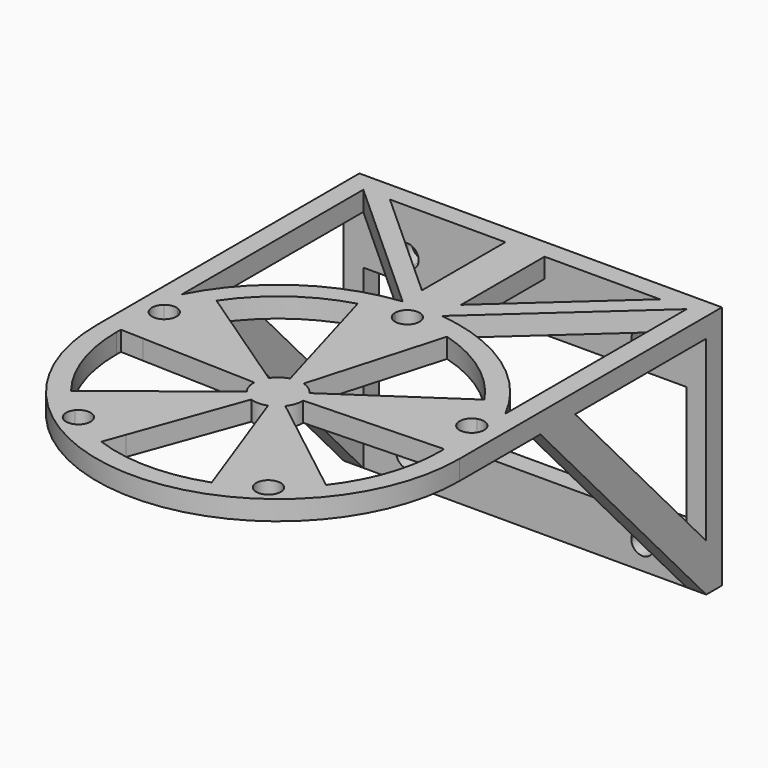
from build123d import *

# Parameters (mm, degrees)
F1_DEPTH = 4
F3_DEPTH = 4
F5_DEPTH = 4
F6_W     = 4
F6_H     = 26
F6_H_2   = 10
F7_DEPTH = 4


with BuildPart() as f1:
    # F0 (on Top) → F1 (new body)
    with BuildSketch(Plane.XY):
        with BuildLine():
            ThreePointArc((-2.498205853, 32.9053030303), (-0.0473569821, 35.499551423), (2.5, 33))
            ThreePointArc((2.5, 33), (2.499551423, 32.9526430179), (2.498205853, 32.9053030303))
            ThreePointArc((2.498205853, 32.9053030303), (5.8372772609, 32.4796273713), (9.1156141969, 31.7160145323))
            ThreePointArc((9.1156141969, 31.7160145323), (19.3969133257, 26.6975608144), (27.3468425908, 18.4702517664))
            ThreePointArc((27.3468425908, 18.4702517664), (29.0861433838, 15.5883374051), (30.5228148036, 12.544232797))
            ThreePointArc((30.5228148036, 12.544232797), (31.8205738268, 12.6592996005), (33, 12.1057901124))
            Line((33, 12.1057901124), (33, 16.7332005307))
            ThreePointArc((33, 16.7332005307), (21.0416278254, 30.4343539188), (4, 36.7831483155))
            ThreePointArc((4, 36.7831483155), (0, 37), (-4, 36.7831483155))
            ThreePointArc((-4, 36.7831483155), (-21.0416278254, 30.4343539188), (-33, 16.7332005307))
            Line((-33, 16.7332005307), (-33, 12.1057901124))
            ThreePointArc((-33, 12.1057901124), (-31.8205738268, 12.6592996005), (-30.5228148036, 12.544232797))
            ThreePointArc((-30.5228148036, 12.544232797), (-29.0861433838, 15.5883374051), (-27.3468425908, 18.4702517664))
            ThreePointArc((-27.3468425908, 18.4702517664), (-19.3969133257, 26.6975608144), (-9.1156141969, 31.7160145323))
            ThreePointArc((-9.1156141969, 31.7160145323), (-5.8372772609, 32.4796273713), (-2.498205853, 32.9053030303))
        make_face()
        with BuildLine():
            ThreePointArc((2.498205853, 32.9053030303), (0, 30.5), (-2.498205853, 32.9053030303))
            ThreePointArc((-2.498205853, 32.9053030303), (-5.8372772609, 32.4796273713), (-9.1156141969, 31.7160145323))
            Line((-9.1156141969, 31.7160145323), (-7.8462162594, 27.2993902036))
            Line((-7.8462162594, 27.2993902036), (-1.3811536662, 4.8054567473))
            ThreePointArc((-1.3811536662, 4.8054567473), (0, 5), (1.3811536662, 4.8054567473))
            Line((1.3811536662, 4.8054567473), (7.8462162594, 27.2993902036))
            Line((7.8462162594, 27.2993902036), (9.1156141969, 31.7160145323))
            ThreePointArc((9.1156141969, 31.7160145323), (5.8372772609, 32.4796273713), (2.498205853, 32.9053030303))
        make_face()
        with BuildLine():
            Line((-4.1434609986, 2.7985229949), (-27.3468425908, 18.4702517664))
            ThreePointArc((-27.3468425908, 18.4702517664), (-29.0861433838, 15.5883374051), (-30.5228148036, 12.544232797))
            ThreePointArc((-30.5228148036, 12.544232797), (-29.3348497225, 11.6284476748), (-28.8848650377, 10.1975608144))
            ThreePointArc((-28.8848650377, 10.1975608144), (-29.8773529706, 8.2032169705), (-32.0667909317, 7.7923628859))
            ThreePointArc((-32.0667909317, 7.7923628859), (-32.6937791328, 4.4851762523), (-32.9806019929, 1.1313232023))
            Line((-32.9806019929, 1.1313232023), (-28.3878771097, 0.9737804072))
            Line((-28.3878771097, 0.9737804072), (-4.997060908, 0.1714126064))
            ThreePointArc((-4.997060908, 0.1714126064), (-4.7552825815, 1.5450849719), (-4.1434609986, 2.7985229949))
        make_face()
        with BuildLine():
            ThreePointArc((30.5228148036, 12.544232797), (29.0861433838, 15.5883374051), (27.3468425908, 18.4702517664))
            Line((27.3468425908, 18.4702517664), (23.5386487783, 15.8981706108))
            Line((23.5386487783, 15.8981706108), (4.1434609986, 2.7985229949))
            ThreePointArc((4.1434609986, 2.7985229949), (4.7552825815, 1.5450849719), (4.997060908, 0.1714126064))
            Line((4.997060908, 0.1714126064), (32.9806019929, 1.1313232023))
            ThreePointArc((32.9806019929, 1.1313232023), (32.6937791328, 4.4851762523), (32.0667909317, 7.7923628859))
            ThreePointArc((32.0667909317, 7.7923628859), (29.007223747, 9.4250183284), (30.5228148036, 12.544232797))
        make_face()
        with BuildLine():
            ThreePointArc((1.3811536662, 4.8054567473), (0, 5), (-1.3811536662, 4.8054567473))
            Line((-1.3811536662, 4.8054567473), (0, 0))
            Line((0, 0), (1.3811536662, 4.8054567473))
        make_face()
        with BuildLine():
            Line((0, 0), (-1.3811536662, 4.8054567473))
            ThreePointArc((-1.3811536662, 4.8054567473), (-2.9389262615, 4.0450849719), (-4.1434609986, 2.7985229949))
            Line((-4.1434609986, 2.7985229949), (0, 0))
        make_face()
        with BuildLine():
            Line((0, 0), (-4.1434609986, 2.7985229949))
            ThreePointArc((-4.1434609986, 2.7985229949), (-4.7552825815, 1.5450849719), (-4.997060908, 0.1714126064))
            Line((-4.997060908, 0.1714126064), (0, 0))
        make_face()
        with BuildLine():
            ThreePointArc((4.1434609986, 2.7985229949), (2.9389262615, 4.0450849719), (1.3811536662, 4.8054567473))
            Line((1.3811536662, 4.8054567473), (0, 0))
            Line((0, 0), (4.1434609986, 2.7985229949))
        make_face()
        with BuildLine():
            Line((-1.7071998188, -4.6995179305), (0, 0))
            Line((0, 0), (-3.9419533944, -3.0758744182))
            ThreePointArc((-3.9419533944, -3.0758744182), (-2.9389262615, -4.0450849719), (-1.7071998188, -4.6995179305))
        make_face()
        with BuildLine():
            Line((-3.9419533944, -3.0758744182), (0, 0))
            Line((0, 0), (-4.997060908, 0.1714126064))
            ThreePointArc((-4.997060908, 0.1714126064), (-4.7552825815, -1.5450849719), (-3.9419533944, -3.0758744182))
        make_face()
        with BuildLine():
            Line((3.9419533944, -3.0758744182), (0, 0))
            Line((0, 0), (1.7071998188, -4.6995179305))
            ThreePointArc((1.7071998188, -4.6995179305), (2.9389262615, -4.0450849719), (3.9419533944, -3.0758744182))
        make_face()
        with BuildLine():
            Line((1.7071998188, -4.6995179305), (0, 0))
            Line((0, 0), (-1.7071998188, -4.6995179305))
            ThreePointArc((-1.7071998188, -4.6995179305), (0, -5), (1.7071998188, -4.6995179305))
        make_face()
        with BuildLine():
            Line((4.1434609986, 2.7985229949), (0, 0))
            Line((0, 0), (4.997060908, 0.1714126064))
            ThreePointArc((4.997060908, 0.1714126064), (4.7552825815, 1.5450849719), (4.1434609986, 2.7985229949))
        make_face()
        with BuildLine():
            Line((4.997060908, 0.1714126064), (0, 0))
            Line((0, 0), (3.9419533944, -3.0758744182))
            ThreePointArc((3.9419533944, -3.0758744182), (4.7280951224, -1.6263814171), (5, 0))
            ThreePointArc((5, 0), (4.999265173, 0.0857189009), (4.997060908, 0.1714126064))
        make_face()
        with BuildLine():
            ThreePointArc((-33, 8.2893315164), (-33.8848650377, 10.1975608144), (-33, 12.1057901124))
            Line((-33, 12.1057901124), (-33, 16.7332005307))
            ThreePointArc((-33, 16.7332005307), (-35.9861084309, 8.602325267), (-37, 0))
            ThreePointArc((-37, 0), (0, -37), (37, 0))
            ThreePointArc((37, 0), (35.9861084309, 8.602325267), (33, 16.7332005307))
            Line((33, 16.7332005307), (33, 12.1057901124))
            ThreePointArc((33, 12.1057901124), (33.6528859157, 11.2492648113), (33.8848650377, 10.1975608144))
            ThreePointArc((33.8848650377, 10.1975608144), (33.6528859157, 9.1458568174), (33, 8.2893315164))
            Line((33, 8.2893315164), (33, 0))
            ThreePointArc((33, 0), (31.2054278075, -10.7341173531), (26.0168924031, -20.3007711599))
            ThreePointArc((26.0168924031, -20.3007711599), (23.8135024738, -22.8455050268), (21.3623428339, -25.152540799))
            ThreePointArc((21.3623428339, -25.152540799), (21.759493882, -25.8801177799), (21.8969133257, -26.6975608144))
            ThreePointArc((21.8969133257, -26.6975608144), (20.1242780272, -29.0894095953), (17.3201608529, -28.0893579142))
            ThreePointArc((17.3201608529, -28.0893579142), (14.3685894638, -29.7076360019), (11.2675188041, -31.016818341))
            ThreePointArc((11.2675188041, -31.016818341), (0, -33), (-11.2675188041, -31.016818341))
            ThreePointArc((-11.2675188041, -31.016818341), (-14.3685894638, -29.7076360019), (-17.3201608529, -28.0893579142))
            ThreePointArc((-17.3201608529, -28.0893579142), (-20.8663764564, -28.7201033003), (-21.3623428339, -25.152540799))
            ThreePointArc((-21.3623428339, -25.152540799), (-23.8135024738, -22.8455050268), (-26.0168924031, -20.3007711599))
            ThreePointArc((-26.0168924031, -20.3007711599), (-31.2054278075, -10.7341173531), (-33, 0))
            Line((-33, 0), (-33, 8.2893315164))
        make_face()
        with BuildLine():
            ThreePointArc((-32.9806019929, 1.1313232023), (-32.6937791328, 4.4851762523), (-32.0667909317, 7.7923628859))
            ThreePointArc((-32.0667909317, 7.7923628859), (-32.5599678414, 7.9909495208), (-33, 8.2893315164))
            Line((-33, 8.2893315164), (-33, 0))
            ThreePointArc((-33, 0), (-32.9951501418, 0.565744746), (-32.9806019929, 1.1313232023))
        make_face()
        with BuildLine():
            ThreePointArc((33, 8.2893315164), (32.5599678414, 7.9909495208), (32.0667909317, 7.7923628859))
            ThreePointArc((32.0667909317, 7.7923628859), (32.6937791328, 4.4851762523), (32.9806019929, 1.1313232023))
            ThreePointArc((32.9806019929, 1.1313232023), (32.9951501418, 0.565744746), (33, 0))
            Line((33, 0), (33, 8.2893315164))
        make_face()
        with BuildLine():
            ThreePointArc((-1.7071998188, -4.6995179305), (-2.9389262615, -4.0450849719), (-3.9419533944, -3.0758744182))
            Line((-3.9419533944, -3.0758744182), (-26.0168924031, -20.3007711599))
            ThreePointArc((-26.0168924031, -20.3007711599), (-23.8135024738, -22.8455050268), (-21.3623428339, -25.152540799))
            ThreePointArc((-21.3623428339, -25.152540799), (-18.5794702912, -24.334980258), (-16.8969133257, -26.6975608144))
            ThreePointArc((-16.8969133257, -26.6975608144), (-17.0050645447, -27.4249255159), (-17.3201608529, -28.0893579142))
            ThreePointArc((-17.3201608529, -28.0893579142), (-14.3685894638, -29.7076360019), (-11.2675188041, -31.016818341))
            Line((-11.2675188041, -31.016818341), (-9.6984566628, -26.6975608144))
            Line((-9.6984566628, -26.6975608144), (-1.7071998188, -4.6995179305))
        make_face()
        with BuildLine():
            ThreePointArc((3.9419533944, -3.0758744182), (2.9389262615, -4.0450849719), (1.7071998188, -4.6995179305))
            Line((1.7071998188, -4.6995179305), (11.2675188041, -31.016818341))
            ThreePointArc((11.2675188041, -31.016818341), (14.3685894638, -29.7076360019), (17.3201608529, -28.0893579142))
            ThreePointArc((17.3201608529, -28.0893579142), (17.9274501949, -24.6750183284), (21.3623428339, -25.152540799))
            ThreePointArc((21.3623428339, -25.152540799), (23.8135024738, -22.8455050268), (26.0168924031, -20.3007711599))
            Line((26.0168924031, -20.3007711599), (22.3939012537, -17.4737804072))
            Line((22.3939012537, -17.4737804072), (3.9419533944, -3.0758744182))
        make_face()
        with BuildLine():
            ThreePointArc((-37, 0), (-35.9861084309, 8.602325267), (-33, 16.7332005307))
            Line((-33, 16.7332005307), (-33, 63))
            Line((-33, 63), (-27.5608655065, 63))
            Line((-27.5608655065, 63), (-4, 63))
            Line((-4, 63), (0, 63))
            Line((0, 63), (4, 63))
            Line((4, 63), (27.5608655065, 63))
            Line((27.5608655065, 63), (33, 63))
            Line((33, 63), (33, 16.7332005307))
            ThreePointArc((33, 16.7332005307), (35.9861084309, 8.602325267), (37, 0))
            Line((37, 0), (37, 67))
            Line((37, 67), (0, 67))
            Line((0, 67), (-37, 67))
            Line((-37, 67), (-37, 0))
        make_face()
        Polygon((-27.5608655065, 63), (-33, 63), (-4, 36.7831483155), (-4, 41.7002856364), align=None)
        with BuildLine():
            Line((-4, 41.7002856364), (-4, 36.7831483155))
            ThreePointArc((-4, 36.7831483155), (0, 37), (4, 36.7831483155))
            Line((4, 36.7831483155), (4, 41.7002856364))
            Line((4, 41.7002856364), (-4, 41.7002856364))
        make_face()
        Polygon((4, 36.7831483155), (33, 63), (27.5608655065, 63), (4, 41.7002856364), align=None)
        Polygon((-4, 63), (-4, 41.7002856364), (4, 41.7002856364), (4, 63), (0, 63), align=None)
    extrude(amount=F1_DEPTH)

    # F2 (on face) → F3 (join)
    with BuildSketch(Plane(origin=(-37, 0, 0), x_dir=(0, -1, 0), z_dir=(-1, 0, 0))):
        Polygon((-17, 0), (-17, 4), (-20.68, 0), align=None)
        Polygon((-17, 4), (-67, 4), (-67, 0), (-63, 0), (-29.5643059095, 0), (-20.68, 0), align=None)
        Polygon((-63, 0), (-67, 0), (-67, -46), (-63, -46), (-63, -36.3431457505), align=None)
        Polygon((-63, -46), (-20.68, 0), (-29.5643059095, 0), (-63, -36.3431457505), align=None)
    extrude(amount=-F3_DEPTH)

    # F4 (on face) → F5 (join)
    with BuildSketch(Plane.YZ.offset(37)):
        Polygon((20.68, 0), (17, 4), (17, 0), align=None)
        Polygon((67, 0), (67, 4), (17, 4), (20.68, 0), (26.6568542495, 0), (29.5643059095, 0), (63, 0), align=None)
        Polygon((67, -46), (67, 0), (63, 0), (63, -36.3431457505), (29.5643059095, 0), (26.6568542495, 0), (20.68, 0), (63, -46), align=None)
    extrude(amount=-F5_DEPTH)

    # F6 (on face) → F7 (join)
    with BuildSketch(Plane(origin=(0, 67, 0), x_dir=(-1, 0, 0), z_dir=(0, 1, 0))):
        with BuildLine():
            Line((-33, -36), (-33, -46))
            Line((-33, -46), (0, -46))
            Line((0, -46), (0, -41))
            Line((0, -41), (-21.7, -41))
            ThreePointArc((-21.7, -41), (-25.6263455967, -42.6263455967), (-24, -38.7))
            Line((-24, -38.7), (-24, -36))
            Line((-24, -36), (-33, -36))
        make_face()
        with Locations((-35, -23)):
            Rectangle(F6_W, F6_H)
        with BuildLine():
            Line((0, -41), (0, -46))
            Line((0, -46), (33, -46))
            Line((33, -46), (33, -36))
            Line((33, -36), (24, -36))
            Line((24, -36), (24, -38.7))
            ThreePointArc((24, -38.7), (25.6263455967, -39.3736544033), (26.3, -41))
            ThreePointArc((26.3, -41), (24, -43.3), (21.7, -41))
            Line((21.7, -41), (0, -41))
        make_face()
        with Locations((35, -41)):
            Rectangle(F6_W, F6_H_2)
        with BuildLine():
            Line((-21.7, -41), (0, -41))
            Line((0, -41), (0, -36))
            Line((0, -36), (-24, -36))
            Line((-24, -36), (-24, -38.7))
            ThreePointArc((-24, -38.7), (-22.3736544033, -39.3736544033), (-21.7, -41))
        make_face()
        with BuildLine():
            Line((0, -36), (0, -41))
            Line((0, -41), (21.7, -41))
            ThreePointArc((21.7, -41), (22.3736544033, -39.3736544033), (24, -38.7))
            Line((24, -38.7), (24, -36))
            Line((24, -36), (0, -36))
        make_face()
        with BuildLine():
            Line((-33, 0), (-33, -10))
            Line((-33, -10), (-24, -10))
            Line((-24, -10), (-24, -7.3))
            ThreePointArc((-24, -7.3), (-25.6263455967, -3.3736544033), (-21.7, -5))
            Line((-21.7, -5), (0, -5))
            Line((0, -5), (0, 0))
            Line((0, 0), (-33, 0))
        make_face()
        Polygon((-37, 4), (-37, 0), (-33, 0), (0, 0), (33, 0), (37, 0), (37, 4), align=None)
        with BuildLine():
            Line((-24, -7.3), (-24, -10))
            Line((-24, -10), (0, -10))
            Line((0, -10), (0, -5))
            Line((0, -5), (-21.7, -5))
            ThreePointArc((-21.7, -5), (-22.3736544033, -6.6263455967), (-24, -7.3))
        make_face()
        with BuildLine():
            Line((24, -10), (33, -10))
            Line((33, -10), (33, 0))
            Line((33, 0), (0, 0))
            Line((0, 0), (0, -5))
            Line((0, -5), (21.7, -5))
            ThreePointArc((21.7, -5), (24, -2.7), (26.3, -5))
            ThreePointArc((26.3, -5), (25.6263455967, -6.6263455967), (24, -7.3))
            Line((24, -7.3), (24, -10))
        make_face()
        with BuildLine():
            Line((0, -5), (0, -10))
            Line((0, -10), (24, -10))
            Line((24, -10), (24, -7.3))
            ThreePointArc((24, -7.3), (22.3736544033, -6.6263455967), (21.7, -5))
            Line((21.7, -5), (0, -5))
        make_face()
    extrude(amount=-F7_DEPTH)


solid = f1.part
